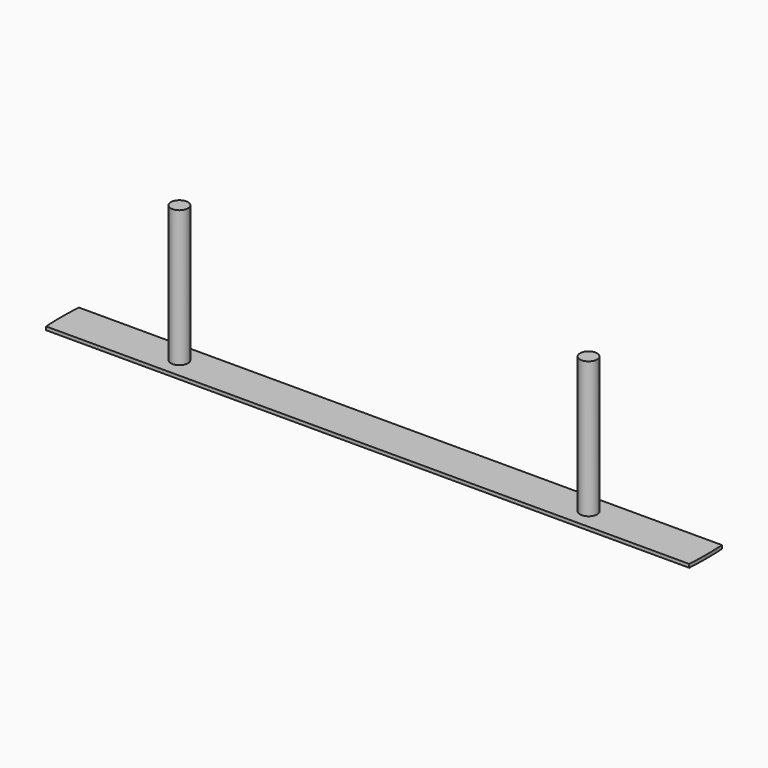
from build123d import *

# Parameters (mm, degrees)
F0_R     = 2.5
F1_DEPTH = 40
F2_DEPTH = 1


# Not quite as in the source:
# - a feature names something its author has since deleted; it is built from what else it names


with BuildPart() as f1:
    # F0 (on Top) → F1 (new body)
    with BuildSketch(Plane.XY):
        with Locations((-60, 0)):
            Circle(F0_R)
    extrude(amount=F1_DEPTH)


with BuildPart() as f1b:
    # F0 (on Top) → F1, piece 2 (new body)
    with BuildSketch(Plane.XY):
        with Locations((60, 0)):
            Circle(F0_R)
    extrude(amount=F1_DEPTH)


with BuildPart() as f2:
    # F0 (on Top) → F2 (new body)
    with BuildSketch(Plane.XY):
        with BuildLine():
            ThreePointArc((94.3093314577, -6), (94.4523208364, -3.0015143883), (94.5, 0))
            ThreePointArc((94.5, 0), (94.4523208364, 3.0015143883), (94.3093314577, 6))
            Line((94.3093314577, 6), (-94.3093314577, 6))
            ThreePointArc((-94.3093314577, 6), (-94.5, 0), (-94.3093314577, -6))
            Line((-94.3093314577, -6), (94.3093314577, -6))
        make_face()
        with Locations((-60, 0)):
            Circle(F0_R, mode=Mode.SUBTRACT)
        with Locations((60, 0)):
            Circle(F0_R, mode=Mode.SUBTRACT)
    extrude(amount=-F2_DEPTH)


solid = Compound([f1.part, f1b.part, f2.part])
